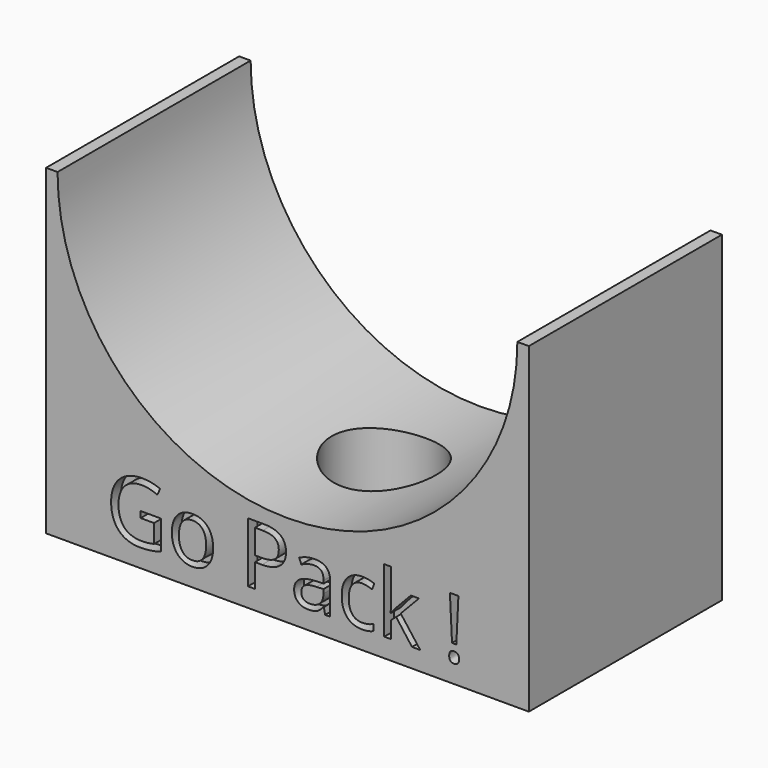
from build123d import *

# Parameters (mm, degrees)
F1_DEPTH       = 30
F3_D           = 9
F3_START       = 8.5750001
F3_CBORE_D     = 13
F3_CBORE_DEPTH = 9
F4_TEXT_SIZE   = 10.4421659166
F5_DEPTH       = 1.5


# Not quite as in the source:
# - Text() gives the source's letters only with a copy of the font that has no kerning and outlines rounded to 1/6400 em; it was checked with that copy


with BuildPart() as f1:
    # F0 (on Front) → F1 (new body)
    with BuildSketch(Plane.XZ):
        with BuildLine():
            Line((-30, -20), (30, -20))
            Line((30, -20), (30, 20))
            Line((30, 20), (28.575, 20))
            ThreePointArc((28.575, 20), (0, -8.575), (-28.575, 20))
            Line((-28.575, 20), (-30, 20))
            Line((-30, 20), (-30, -20))
        make_face()
    extrude(amount=F1_DEPTH)

    # F3 (through all)
    # its depths count from where the whole tool has entered the part; down to there all is cleared
    with Locations(Plane.XY.offset(-F3_START)):
        with Locations((0, -15)):
            CounterBoreHole(F3_D / 2, F3_CBORE_D / 2, F3_CBORE_DEPTH)

    # F4 (on face) → F5 (cut)
    with BuildSketch(Plane.XZ.offset(30)):
        with Locations((-22.5550811738, -17.6392290741)):
            Text('Go Pack !', F4_TEXT_SIZE, font='Open Sans', text_align=(TextAlign.LEFT, TextAlign.BOTTOM))
    extrude(amount=-F5_DEPTH, mode=Mode.SUBTRACT)


solid = f1.part
